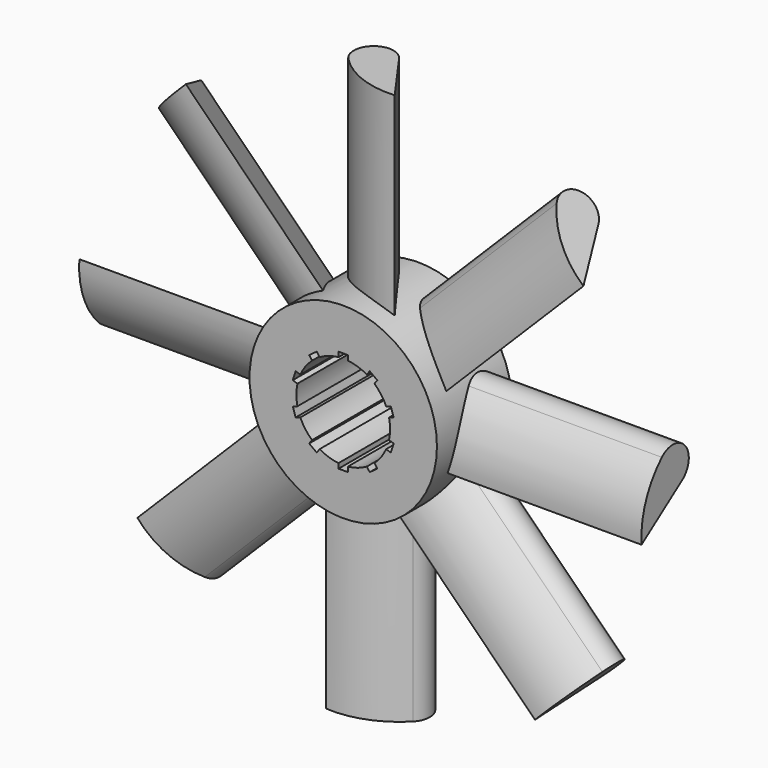
from build123d import *

# Parameters (mm, degrees)
F0_R            = 12.7
F0_R_2          = 6.35
F1_DEPTH        = 6.35
F4_DEPTH        = 25.4
F7_DEPTH        = 30.48
F7_COPIES_COUNT = 8


# Not quite as in the source:
# - a pattern or mirror of a feature is missing from the dataset's text; its kind, count and spacing are read off the source's solid


with BuildPart() as f1:
    # F0 (on Front) → F1 (new body, symmetric)
    with BuildSketch(Plane.XZ):
        Circle(F0_R)
        Circle(F0_R_2, mode=Mode.SUBTRACT)
    extrude(amount=F1_DEPTH, both=True)

    # F3 (on offset) → F4 (cut)
    with BuildSketch(Plane.XZ.offset(6.35)):
        with BuildLine():
            Line((-3.2000014887, 5.4847507211), (-3.5919541958, 6.0242273409))
            Line((-3.5919541958, 6.0242273409), (-4.6194057787, 5.2777400705))
            Line((-4.6194057787, 5.2777400705), (-4.2274530715, 4.7382634507))
            ThreePointArc((-4.2274530715, 4.7382634507), (-3.7324363521, 5.1372579143), (-3.2000014887, 5.4847507211))
        make_face()
        with BuildLine():
            ThreePointArc((-0.635, 6.3181702256), (0, 6.35), (0.635, 6.3181702256))
            Line((0.635, 6.3181702256), (0.635, 6.985))
            Line((0.635, 6.985), (-0.635, 6.985))
            Line((-0.635, 6.985), (-0.635, 6.3181702256))
        make_face()
        with BuildLine():
            Line((4.2274530715, 4.7382634507), (4.6194057787, 5.2777400705))
            Line((4.6194057787, 5.2777400705), (3.5919541958, 6.0242273409))
            Line((3.5919541958, 6.0242273409), (3.2000014887, 5.4847507211))
            ThreePointArc((3.2000014887, 5.4847507211), (3.7324363521, 5.1372579143), (4.2274530715, 4.7382634507))
        make_face()
        with BuildLine():
            Line((6.2051627556, 1.3485010852), (6.8393555577, 1.5545628179))
            Line((6.8393555577, 1.5545628179), (6.4469039749, 2.7624045936))
            Line((6.4469039749, 2.7624045936), (5.8127111727, 2.5563428609))
            ThreePointArc((5.8127111727, 2.5563428609), (6.0392088785, 1.9622579143), (6.2051627556, 1.3485010852))
        make_face()
        with BuildLine():
            Line((5.8127111727, -2.5563428609), (6.4469039749, -2.7624045936))
            Line((6.4469039749, -2.7624045936), (6.8393555577, -1.5545628179))
            Line((6.8393555577, -1.5545628179), (6.2051627556, -1.3485010852))
            ThreePointArc((6.2051627556, -1.3485010852), (6.0392088785, -1.9622579143), (5.8127111727, -2.5563428609))
        make_face()
        with BuildLine():
            Line((-6.2051627556, -1.3485010852), (-6.8393555577, -1.5545628179))
            Line((-6.8393555577, -1.5545628179), (-6.4469039749, -2.7624045936))
            Line((-6.4469039749, -2.7624045936), (-5.8127111727, -2.5563428609))
            ThreePointArc((-5.8127111727, -2.5563428609), (-6.0392088785, -1.9622579143), (-6.2051627556, -1.3485010852))
        make_face()
        with BuildLine():
            Line((-5.8127111727, 2.5563428609), (-6.4469039749, 2.7624045936))
            Line((-6.4469039749, 2.7624045936), (-6.8393555577, 1.5545628179))
            Line((-6.8393555577, 1.5545628179), (-6.2051627556, 1.3485010852))
            ThreePointArc((-6.2051627556, 1.3485010852), (-6.0392088785, 1.9622579143), (-5.8127111727, 2.5563428609))
        make_face()
        with BuildLine():
            Line((-4.2274530715, -4.7382634507), (-4.6194057787, -5.2777400705))
            Line((-4.6194057787, -5.2777400705), (-3.5919541958, -6.0242273409))
            Line((-3.5919541958, -6.0242273409), (-3.2000014887, -5.4847507211))
            ThreePointArc((-3.2000014887, -5.4847507211), (-3.7324363521, -5.1372579143), (-4.2274530715, -4.7382634507))
        make_face()
        with BuildLine():
            Line((-0.635, -6.3181702256), (-0.635, -6.985))
            Line((-0.635, -6.985), (0.635, -6.985))
            Line((0.635, -6.985), (0.635, -6.3181702256))
            ThreePointArc((0.635, -6.3181702256), (0, -6.35), (-0.635, -6.3181702256))
        make_face()
        with BuildLine():
            Line((3.2000014887, -5.4847507211), (3.5919541958, -6.0242273409))
            Line((3.5919541958, -6.0242273409), (4.6194057787, -5.2777400705))
            Line((4.6194057787, -5.2777400705), (4.2274530715, -4.7382634507))
            ThreePointArc((4.2274530715, -4.7382634507), (3.7324363521, -5.1372579143), (3.2000014887, -5.4847507211))
        make_face()
    extrude(amount=-F4_DEPTH, mode=Mode.SUBTRACT)

    # F6 (on offset) → F7 (join)
    with BuildSketch(Plane.YZ.offset(38.1)):
        with BuildLine():
            ThreePointArc((0, 4.386866935), (-2.7218067049, 0.2512213266), (-3.4407728063, -4.64723599))
            Line((-3.4407728063, -4.64723599), (3.4407728063, 0.260369055))
            ThreePointArc((3.4407728063, 0.260369055), (3.9456637131, 4.1791075354), (0, 4.386866935))
        make_face()
    f7 = extrude(amount=-F7_DEPTH)

    # F7_copies: F7 ×8 about axis
    f7_copies_axis = Axis((0, 0, 0), (0, 1, 0))
    for i in range(1, F7_COPIES_COUNT):
        add(f7.rotate(f7_copies_axis, i * 360 / F7_COPIES_COUNT))


solid = f1.part
